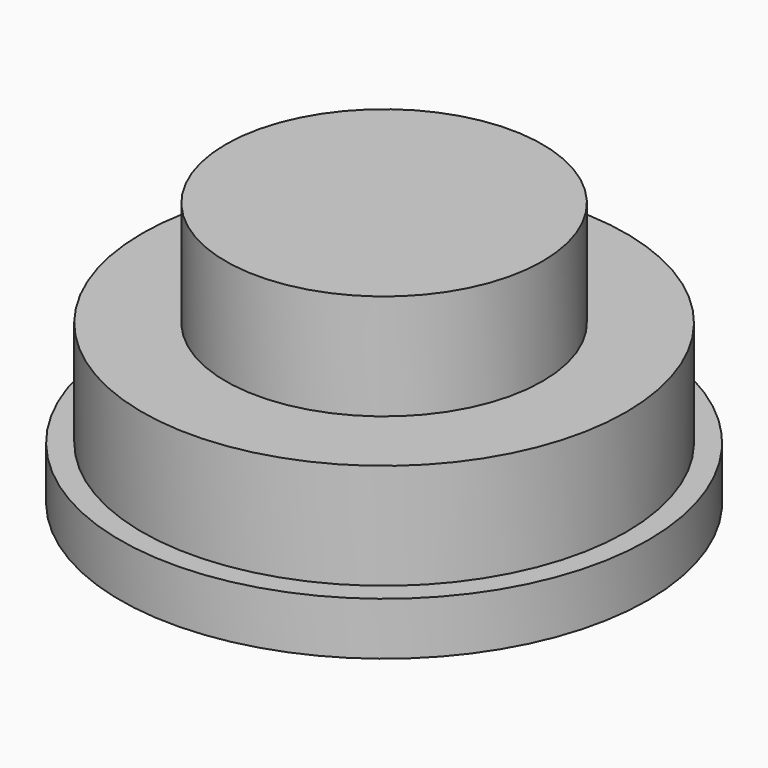
from build123d import *

# Parameters (mm, degrees)
F0_R     = 50.8
F1_DEPTH = 10.16
F2_R     = 46.5709
F3_DEPTH = 20.32
F4_R     = 30.48
F5_DEPTH = 20.32


# Not quite as in the source:
# - a feature names something its author has since deleted; it is built from what else it names


with BuildPart() as f1:
    # F0 (on Top) → F1 (new body)
    with BuildSketch(Plane.XY):
        Circle(F0_R)
    extrude(amount=F1_DEPTH)

    # F2 (on face) → F3 (join)
    with BuildSketch(Plane.XY.offset(10.16)):
        Circle(F2_R)
    extrude(amount=F3_DEPTH)

    # F4 (on face) → F5 (join)
    with BuildSketch(Plane.XY.offset(30.48)):
        Circle(F4_R)
    extrude(amount=F5_DEPTH)


solid = f1.part
